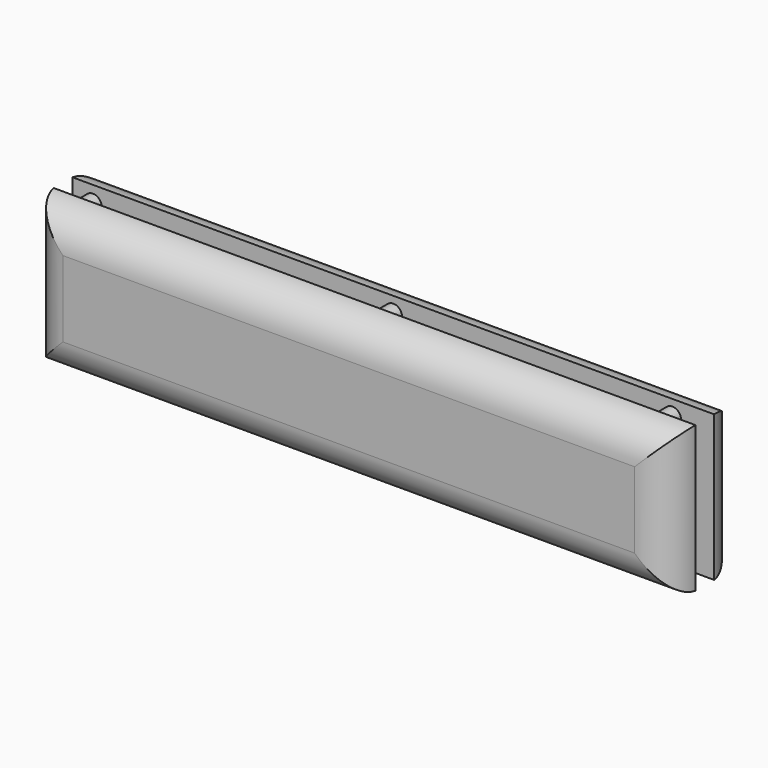
from build123d import *

# Parameters (mm, degrees)
F0_W        = 110
F0_H        = 25
F1_DEPTH    = 5.55
F2_R        = 2
F3_DEPTH    = 2
F4_R        = 1.5
F5_DEPTH    = 1
F6_DEPTH    = 2
F8_T1_DEPTH = 139.9155060128
F8_T3_DEPTH = 54.9155060128


# Not quite as in the source:
# - a fillet or chamfer that OpenCascade refuses, or shapes differently, is made with other operations: its cross-section is extruded or revolved along the edge and cut away or added


with BuildPart() as f1:
    # F0 (on Front) → F1 (new body)
    with BuildSketch(Plane.XZ):
        Rectangle(F0_W, F0_H)
    extrude(amount=F1_DEPTH)

    # F2 (on face) → F3 (cut)
    with BuildSketch(Plane.XZ.offset(5.55)):
        with Locations((-49, 0)):
            Circle(F2_R)
    extrude(amount=-F3_DEPTH, mode=Mode.SUBTRACT)

    # F4 (on face) → F5 (join)
    with BuildSketch(Plane.XZ.offset(5.55)):
        with Locations((0, 9.82276164)):
            Circle(F4_R)
        with Locations((-51.5013597906, 9.6743786708)):
            Circle(F4_R)
        with Locations((47.8420853615, 9.8438328132)):
            Circle(F4_R)
    extrude(amount=F5_DEPTH)

    # F4 (on face) → F6 (join)
    with BuildSketch(Plane.XZ.offset(5.55)):
        with Locations((0, 9.82276164)):
            Circle(F4_R)
        with Locations((-51.5013597906, 9.6743786708)):
            Circle(F4_R)
        with Locations((47.8420853615, 9.8438328132)):
            Circle(F4_R)
    extrude(amount=F6_DEPTH)

    # F7: F1 across face


with BuildPart() as f1_1:
    add(f1.part)
    add(f1.part.mirror(Plane(origin=(0, -7.55, 9.82276164), x_dir=(1, 0, 0), z_dir=(0, -1, 0))))

    # F8: fillet of radius 6 on 8 edges, made by hand

    # F8_s2 → F8_t1 (cut)
    with BuildSketch(Plane.YZ.offset(-69.9577530064)):
        with BuildLine():
            ThreePointArc((-9.55, -12.5), (-13.4988634896, -10.5973399501), (-15.1, -6.5168987974))
            Line((-15.1, -6.5168987974), (-15.1, -12.5))
            Line((-15.1, -12.5), (-9.55, -12.5))
        make_face()
        with BuildLine():
            ThreePointArc((-9.55, 12.5), (-13.4988634896, 10.5973399501), (-15.1, 6.5168987974))
            Line((-15.1, 6.5168987974), (-15.1, 12.5))
            Line((-15.1, 12.5), (-9.55, 12.5))
        make_face()
        with BuildLine():
            ThreePointArc((-5.55, -12.5), (-1.6011365104, -10.5973399501), (0, -6.5168987974))
            Line((0, -6.5168987974), (0, -12.5))
            Line((0, -12.5), (-5.55, -12.5))
        make_face()
        with BuildLine():
            ThreePointArc((0, 6.5168987974), (-1.6011365104, 10.5973399501), (-5.55, 12.5))
            Line((-5.55, 12.5), (0, 12.5))
            Line((0, 12.5), (0, 6.5168987974))
        make_face()
    extrude(amount=F8_T1_DEPTH, mode=Mode.SUBTRACT)

    # F8_s4 → F8_t3 (cut)
    with BuildSketch(Plane.XY.offset(-27.4577530064)):
        with BuildLine():
            ThreePointArc((55, -9.55), (53.0973399501, -13.4988634896), (49.0168987974, -15.1))
            Line((49.0168987974, -15.1), (55, -15.1))
            Line((55, -15.1), (55, -9.55))
        make_face()
        with BuildLine():
            ThreePointArc((-55, -9.55), (-53.0973399501, -13.4988634896), (-49.0168987974, -15.1))
            Line((-49.0168987974, -15.1), (-55, -15.1))
            Line((-55, -15.1), (-55, -9.55))
        make_face()
        with BuildLine():
            ThreePointArc((55, -5.55), (53.0973399501, -1.6011365104), (49.0168987974, 0))
            Line((49.0168987974, 0), (55, 0))
            Line((55, 0), (55, -5.55))
        make_face()
        with BuildLine():
            ThreePointArc((-55, -5.55), (-53.0973399501, -1.6011365104), (-49.0168987974, 0))
            Line((-49.0168987974, 0), (-55, 0))
            Line((-55, 0), (-55, -5.55))
        make_face()
    extrude(amount=F8_T3_DEPTH, mode=Mode.SUBTRACT)


solid = f1_1.part
